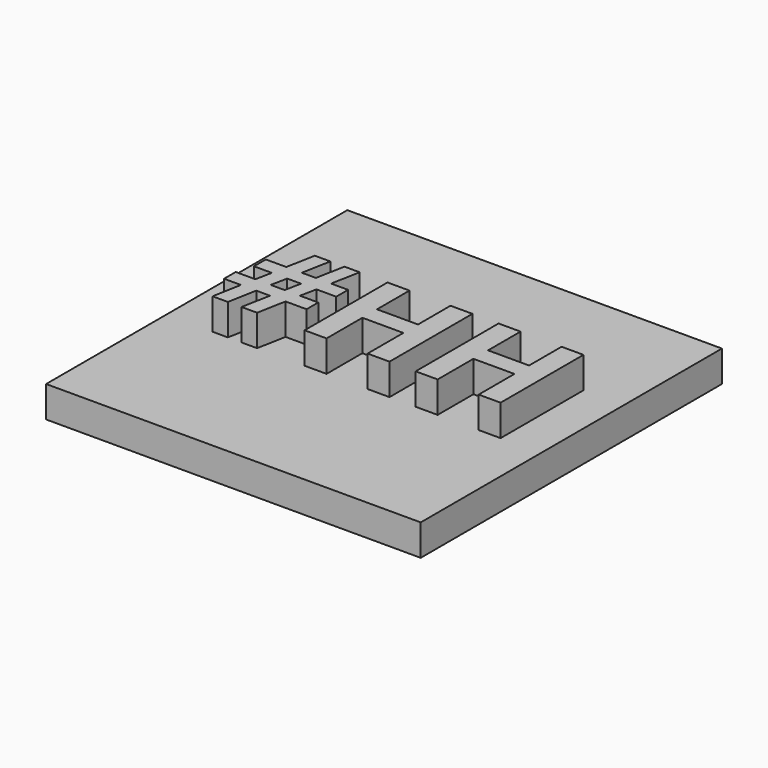
from build123d import *

# Parameters (mm, degrees)
F0_W         = 152.4
F0_H         = 153.1667833941
F1_DEPTH     = 12.7
F2_TEXT_SIZE = 59.0483109335
F3_DEPTH     = 12.7


# Not quite as in the source:
# - Text() gives the source's letters only with a copy of the font that has no kerning and outlines rounded to 1/6400 em; it was checked with that copy


with BuildPart() as f1:
    # F0 (on Top) → F1 (new body)
    with BuildSketch(Plane.XY):
        Rectangle(F0_W, F0_H)
    extrude(amount=F1_DEPTH)

    # F2 (on face) → F3 (join)
    with BuildSketch(Plane.XY.offset(12.7)):
        with Locations((-63.3637189553, -15.4792772737)):
            Text('#HH', F2_TEXT_SIZE, font='Open Sans', font_style=FontStyle.BOLD, text_align=(TextAlign.LEFT, TextAlign.BOTTOM))
    extrude(amount=F3_DEPTH)


solid = f1.part
